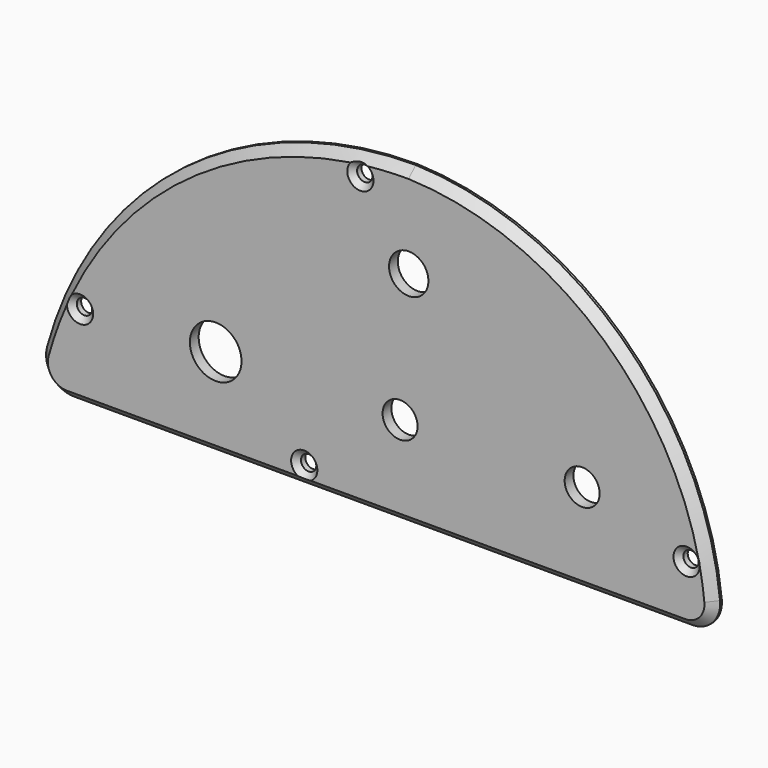
from build123d import *

# Parameters (mm, degrees)
F1_DEPTH       = 2.5
F2_D           = 3.5
F2_CSINK_D     = 6
F2_CSINK_ANGLE = 90
F3_T1_DEPTH    = 141.3928063628
F3_T4_ANGLE    = 86.5781008802
F3_T6_ANGLE    = 95.6855323437
F3_T8_ANGLE    = 105.4133416791
F3_T10_ANGLE   = 78.1582231343
F4_D           = 11.8
F5_D           = 8
F6_D           = 9


# Not quite as in the source:
# - a fillet or chamfer that OpenCascade refuses, or shapes differently, is made with other operations: its cross-section is extruded or revolved along the edge and cut away or added


with BuildPart() as f1:
    # F0 (on Front) → F1 (new body)
    with BuildSketch(Plane.XZ):
        with BuildLine():
            ThreePointArc((51.9193532242, 6.9790848915), (29.3726830737, 52.5798387856), (-17.6447437911, 72))
            ThreePointArc((-17.6447437911, 72), (-70.6003478325, 54.2753932247), (-101.9138280482, 8.0377068475))
            ThreePointArc((-101.9138280482, 8.0377068475), (-100.843919646, 2.5025617927), (-95.7922150584, 0))
            Line((-95.7922150584, 0), (45.6005913044, 0))
            ThreePointArc((45.6005913044, 0), (50.3078829387, 2.0880866422), (51.9193532242, 6.9790848915))
        make_face()
    extrude(amount=-F1_DEPTH)

    # F2 (through all)
    with Locations(Plane.XZ):
        with Locations((-92.7765071392, 19.3704143167), (-28.6957714707, 67.0258700848), (45.8813235164, 13.6932386085), (-41.5233448148, 4.6045258641)):
            CounterSinkHole(F2_D / 2, F2_CSINK_D / 2, counter_sink_angle=F2_CSINK_ANGLE)

    # F3: chamfer of 2 on 1 edges, made by hand

    # F3_s2 → F3_t1 (cut)
    with BuildSketch(Plane.YZ.offset(-95.7922150584)):
        Polygon((0, 2), (2, 0), (0, 0), align=None)
    extrude(amount=F3_T1_DEPTH, mode=Mode.SUBTRACT)

    # F3_s3 → F3_t4 (revolve, cut)
    with BuildSketch(Plane(origin=(-0.1784402108, 0, 1.7923196444), x_dir=(0, 1, 0), z_dir=(0.0990684869, 0, -0.9950806173))):
        Polygon((2, 52.3553494356), (0, 50.3553494356), (0, 52.3553494356), align=None)
    revolve(axis=Axis((-19.9365535802, 0, -0.1747635854), (0, -1, 0)), revolution_arc=F3_T4_ANGLE, mode=Mode.SUBTRACT)

    # F3_s5 → F3_t6 (revolve, cut)
    with BuildSketch(Plane.YZ.offset(45.6005913044)):
        Polygon((2, 0), (0, 2), (0, 0), align=None)
    revolve(axis=Axis((45.6005913044, 0, 6.35), (0, -1, 0)), revolution_arc=F3_T6_ANGLE, mode=Mode.SUBTRACT)

    # F3_s7 → F3_t8 (revolve, cut)
    with BuildSketch(Plane(origin=(-5.1396919269, 0, -18.6425770032), x_dir=(0, 1, 0), z_dir=(0.2657806059, 0, 0.9640335417))):
        Polygon((0, 98.3846151976), (2, 100.3846151976), (0, 100.3846151976), align=None)
    revolve(axis=Axis((-95.7922150584, 0, 6.35), (0, -1, 0)), revolution_arc=F3_T8_ANGLE, mode=Mode.SUBTRACT)

    # F3_s9 → F3_t10 (revolve, cut)
    with BuildSketch(Plane(origin=(-16.9209977533, 0, 1.0561482837), x_dir=(0, 1, 0), z_dir=(0.9980577677, 0, -0.0622952035))):
        Polygon((2, 70.9128484948), (0, 68.9128484948), (0, 70.9128484948), align=None)
    revolve(axis=Axis((-17.9304192048, 0, -15.1162191548), (0, -1, 0)), revolution_arc=F3_T10_ANGLE, mode=Mode.SUBTRACT)

    # F4 (through all)
    with Locations(Plane.XZ):
        with Locations((-61.7667548358, 20.886823535)):
            Hole(F4_D / 2)

    # F5 (through all)
    with Locations(Plane.XZ):
        with Locations((-19.6185931563, 20.886823535), (22.0020785928, 20.886823535)):
            Hole(F5_D / 2)

    # F6 (through all)
    with Locations(Plane.XZ):
        with Locations((-17.6447437911, 50.9389452636)):
            Hole(F6_D / 2)


solid = f1.part
